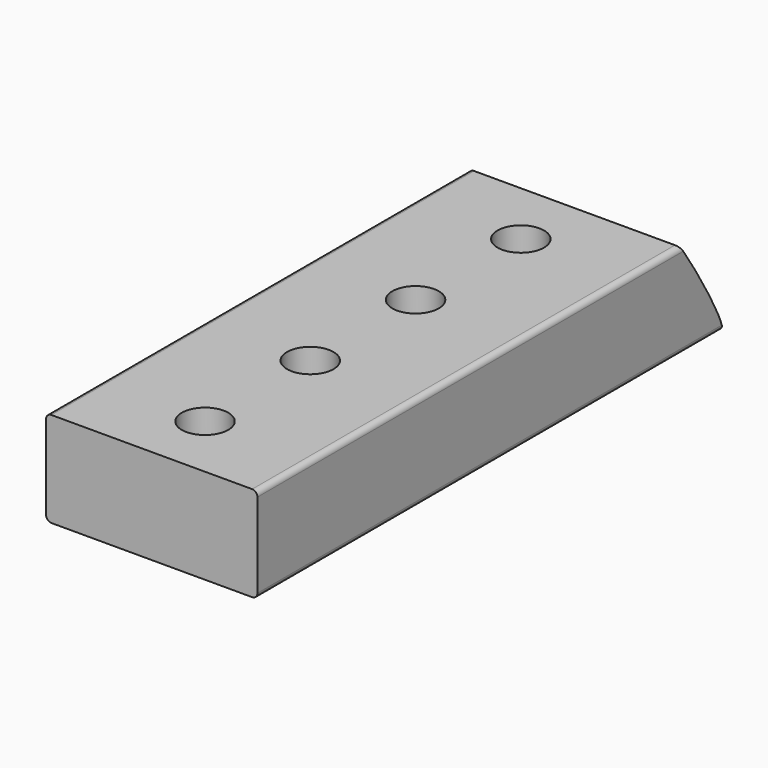
from build123d import *

# Parameters (mm, degrees)
F1_DEPTH = 40
F2_R     = 4.4
F3_DEPTH = 18
F4_R     = 1
F5_R     = 1
F6_DEPTH = 15


with BuildPart() as f1:
    # F0 (on Right) → F1 (new body)
    with BuildSketch(Plane.YZ):
        with BuildLine():
            Line((0, 0), (0, -18))
            Line((0, -18), (108.1519347629, -18))
            Line((108.1519347629, -18), (110, -18))
            add(Edge.make_bspline(
                [(100, 0), (102.15, -2.75), (110.3054567735, -15.7496706799), (110, -18)],
                knots=[0, 0, 0, 0, 0.5188602886, 0.5188602886, 0.5188602886, 0.5188602886], degree=3))
            Line((100, 0), (0, 0))
        make_face()
    extrude(amount=F1_DEPTH)

    # F2 (on face) → F3 (cut, through all)
    with BuildSketch(Plane.XY):
        with Locations((20, 87.3)):
            Circle(F2_R)
        with Locations((20, 62.4)):
            Circle(F2_R)
        with Locations((20, 37.5)):
            Circle(F2_R)
        with Locations((20, 12.6)):
            Circle(F2_R)
    extrude(amount=-F3_DEPTH, mode=Mode.SUBTRACT)

    # F4
    f4_edges = [f1.edges().sort_by_distance(p)[0] for p in [
        (0, 50, 0),
        (0, 55, -18),
        (40, 50, 0),
        (40, 55, -18),
    ]]
    fillet(f4_edges, radius=F4_R)

    # F5 (on face) → F6 (cut)
    with BuildSketch(Plane(origin=(0, 0, -18), x_dir=(1, 0, 0), z_dir=(0, 0, -1))):
        with Locations((20, -72.9)):
            Circle(F5_R)
        with Locations((20, -29)):
            Circle(F5_R)
    extrude(amount=-F6_DEPTH, mode=Mode.SUBTRACT)


solid = f1.part
